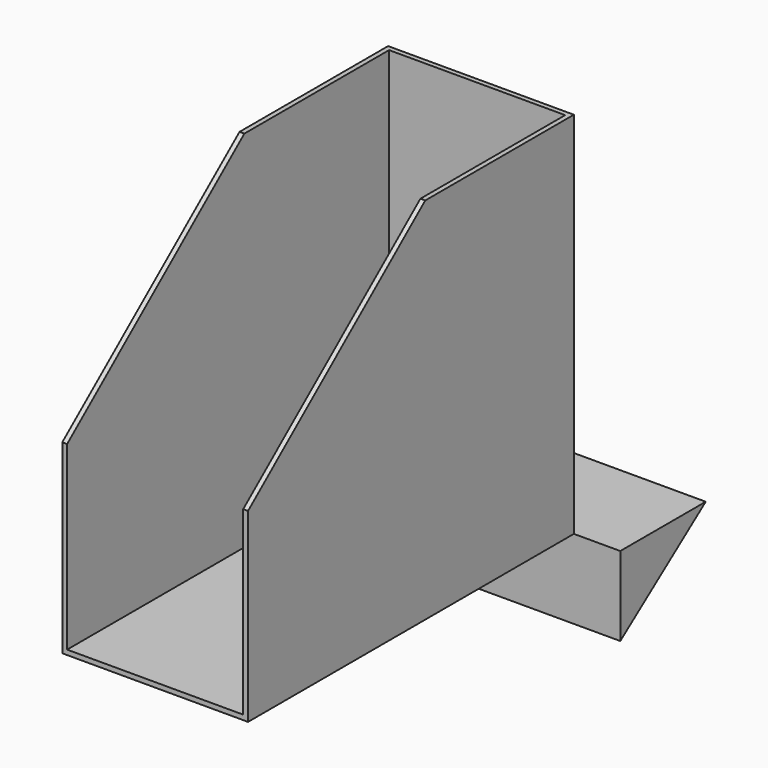
from build123d import *

# Parameters (mm, degrees)
F1_DEPTH = 25
F2_DEPTH = 100
F3_DEPTH = 25
F4_T     = -2.6


with BuildPart() as f1:
    # F0 (on Right) → F1 (new body)
    with BuildSketch(Plane.YZ):
        Polygon((-122.6000512926, 42.5921416433), (-122.6000512926, -57.4078583567), (96.6418987055, -57.4078583567), (96.6418987055, 141.2506547058), (-3.3581012945, 141.2506547058), align=None)
    extrude(amount=F1_DEPTH)

    # F0 (on Right) → F2 (join)
    with BuildSketch(Plane.YZ):
        Polygon((-122.6000512926, 42.5921416433), (-122.6000512926, -57.4078583567), (96.6418987055, -57.4078583567), (96.6418987055, 141.2506547058), (-3.3581012945, 141.2506547058), align=None)
    extrude(amount=F2_DEPTH)

    # F4
    f4_openings = [f1.faces().sort_by_distance(p)[0] for p in [
        (50, 46.641899, 141.250655),
        (50, -62.979076, 91.921398),
        (50, -122.600051, -7.407858),
    ]]
    offset(amount=F4_T, openings=f4_openings)


with BuildPart() as f2:
    # F0 (on Right) → F2, piece 2 (new body)
    with BuildSketch(Plane.YZ):
        Polygon((154.1335378966, -57.4078583567), (96.6418987055, -57.4078583567), (96.6418987055, -100.0723155335), align=None)
    extrude(amount=F2_DEPTH)

    # F3 (add): a face of the model
    f3_faces = [f2.faces().sort_by_distance(p)[0] for p in [
        (100, 115.8057784359, -71.6293440823),
    ]]
    extrude(f3_faces, amount=F3_DEPTH)


solid = Compound([f1.part, f2.part])
